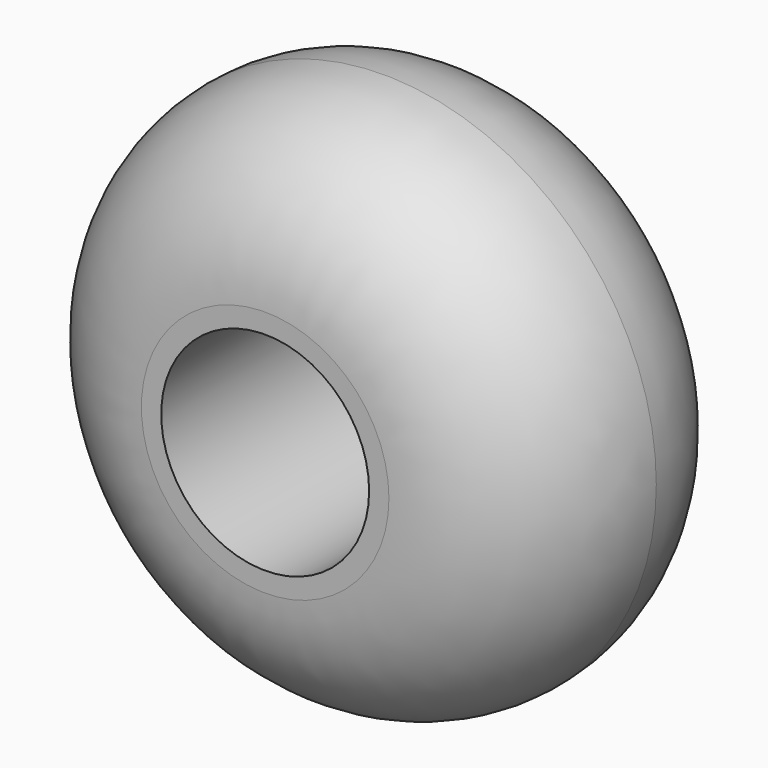
from build123d import *

# Parameters (mm, degrees)
F0_R     = 5.5
F0_R_2   = 2.1
F1_DEPTH = 6
F2_R     = 2.99999


# Not quite as in the source:
# - a fillet or chamfer is up to 0.001 mm smaller than in the source, because OpenCascade refuses the exact size


with BuildPart() as f1:
    # F0 (on Front) → F1 (new body)
    with BuildSketch(Plane.XZ):
        with Locations((0, 2.5408205111)):
            Circle(F0_R)
        with Locations((0, 2.5408205111)):
            Circle(F0_R_2, mode=Mode.SUBTRACT)
    extrude(amount=F1_DEPTH)

    # F2 (radius 3 in the source; OpenCascade refuses exactly that, so slightly less here)
    f2_edges = [f1.edges().sort_by_distance(p)[0] for p in [
        (-5.5, -6, 2.540821),
        (-5.5, 0, 2.540821),
    ]]
    fillet(f2_edges, radius=F2_R)


solid = f1.part
